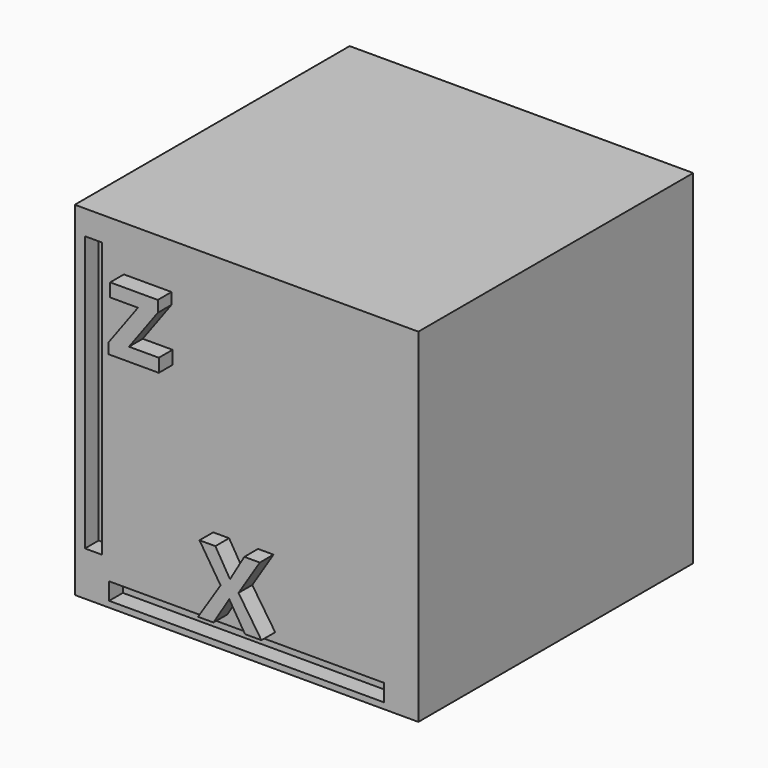
from build123d import *

# Parameters (mm, degrees)
F0_W           = 20
F0_H           = 20
F1_DEPTH       = 20
F2_W           = 1
F2_H           = 16
F2_W_2         = 16
F2_H_2         = 1
F4_DEPTH       = 1
F3_W           = 16
F3_H           = 1
F5_DEPTH       = 1
F3_TEXT_SIZE   = 5.777607152
F6_DEPTH       = 1
F2_TEXT_SIZE   = 6.8080042385
F2_TEXT_SIZE_2 = 5.5314282644
F7_DEPTH       = 1


# Not quite as in the source:
# - Text() gives the source's letters only with a copy of the font that has no kerning and outlines rounded to 1/6400 em; it was checked with that copy


with BuildPart() as f1:
    # F0 (on Top) → F1 (new body)
    with BuildSketch(Plane.XY):
        Rectangle(F0_W, F0_H)
    extrude(amount=F1_DEPTH)

    # F2 (on face) → F4 (cut)
    with BuildSketch(Plane.XZ.offset(10)):
        with Locations((-8.9074783847, 10.5787586346)):
            Rectangle(F2_W, F2_H)
        with Locations((0, 0.852760708)):
            Rectangle(F2_W_2, F2_H_2)
    extrude(amount=-F4_DEPTH, mode=Mode.SUBTRACT)

    # F3 (on face) → F5 (cut)
    with BuildSketch(Plane(origin=(-10, 0, 0), x_dir=(0, -1, 0), z_dir=(-1, 0, 0))):
        with Locations((0, 0.9796705907)):
            Rectangle(F3_W, F3_H)
    extrude(amount=-F5_DEPTH, mode=Mode.SUBTRACT)

    # F3 (on face) → F6 (join)
    with BuildSketch(Plane(origin=(-10, 0, 0), x_dir=(0, -1, 0), z_dir=(-1, 0, 0))):
        with Locations((-1.9901148385, 2.1823853459)):
            Text('Y', F3_TEXT_SIZE, font='Open Sans', font_style=FontStyle.BOLD, text_align=(TextAlign.LEFT, TextAlign.BOTTOM))
    extrude(amount=F6_DEPTH)

    # F2 (on face) → F7 (join)
    with BuildSketch(Plane.XZ.offset(10)):
        with Locations((-7.4269713368, 13.6429527774)):
            Text('z', F2_TEXT_SIZE, font='Open Sans', font_style=FontStyle.BOLD, text_align=(TextAlign.LEFT, TextAlign.BOTTOM))
        with Locations((-2.0241570305, 1.8837660861)):
            Text('X', F2_TEXT_SIZE_2, font='Open Sans', font_style=FontStyle.BOLD, text_align=(TextAlign.LEFT, TextAlign.BOTTOM))
    extrude(amount=F7_DEPTH)


solid = f1.part
